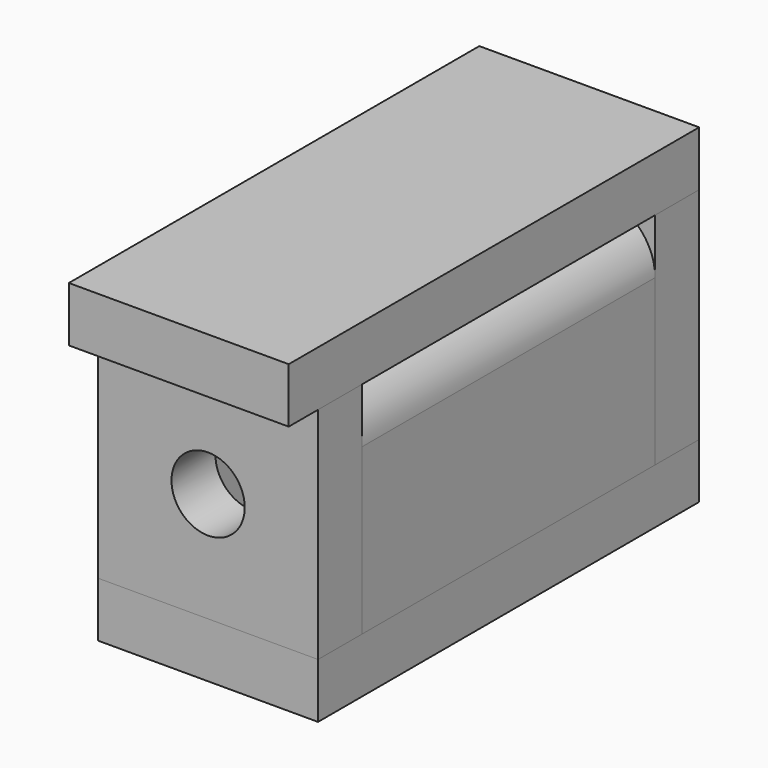
from build123d import *

# Parameters (mm, degrees)
F2_DEPTH  = 38.1
F1_W      = 19.05
F1_H      = 76.2
F3_DEPTH  = 38.1
F4_DEPTH  = 38.1
F5_DEPTH  = 38.1
F6_R      = 12.7
F7_DEPTH  = 19.05
F8_W      = 127
F8_H      = 76.2
F9_DEPTH  = 19.05
F10_W     = 127
F10_H     = 76.2
F11_DEPTH = 19.05
F12_R     = 19.04999


# Not quite as in the source:
# - a variable given as a bare number and used for a length is read in inches; the dataset says mm whatever the document's units were
# - a fillet or chamfer is up to 0.001 mm smaller than in the source, because OpenCascade refuses the exact size
# - a feature names something its author has since deleted; it is built from what else it names


with BuildPart() as f2:
    # F1 (on Right) → F2 (new body, symmetric)
    with BuildSketch(Plane.YZ):
        Polygon((82.55, 0), (82.55, 19.05), (63.5, 19.05), (-63.5, 19.05), (-82.55, 19.05), (-82.55, 0), align=None)
    extrude(amount=F2_DEPTH, both=True)


with BuildPart() as f3:
    # F1 (on Right) → F3 (new body, symmetric)
    with BuildSketch(Plane.YZ):
        with Locations((73.025, 57.15)):
            Rectangle(F1_W, F1_H)
    extrude(amount=F3_DEPTH, both=True)


with BuildPart() as f4:
    # F1 (on Right) → F4 (new body, symmetric)
    with BuildSketch(Plane.YZ):
        Polygon((82.55, 114.3), (-95.25, 114.3), (-95.25, 95.25), (-82.55, 95.25), (-63.5, 95.25), (63.5, 95.25), (82.55, 95.25), align=None)
    extrude(amount=F4_DEPTH, both=True)


with BuildPart() as f5:
    # F1 (on Right) → F5 (new body, symmetric)
    with BuildSketch(Plane.YZ):
        with Locations((-73.025, 57.15)):
            Rectangle(F1_W, F1_H)
    extrude(amount=F5_DEPTH, both=True)

    # F6 (on face) → F7 (cut, through all)
    with BuildSketch(Plane.XZ.offset(82.55)):
        with Locations((0, 57.15)):
            Circle(F6_R)
    extrude(amount=-F7_DEPTH, mode=Mode.SUBTRACT)


with BuildPart() as f9:
    # F8 (on face) → F9 (new body)
    with BuildSketch(Plane(origin=(-38.1, 0, 0), x_dir=(0, -1, 0), z_dir=(-1, 0, 0))):
        with Locations((0, 57.15)):
            Rectangle(F8_W, F8_H)
    extrude(amount=-F9_DEPTH)


with BuildPart() as f11:
    # F10 (on face) → F11 (new body)
    with BuildSketch(Plane.YZ.offset(38.1)):
        with Locations((0, 57.15)):
            Rectangle(F10_W, F10_H)
    extrude(amount=-F11_DEPTH)

    # F12 (radius 19.05 in the source; OpenCascade refuses exactly that, so slightly less here)
    f12_edges = [f11.edges().sort_by_distance(p)[0] for p in [
        (38.1, 0, 95.25),
        (19.05, 0, 19.05),
    ]]
    fillet(f12_edges, radius=F12_R)


solid = Compound([f2.part, f3.part, f4.part, f5.part, f9.part, f11.part])
